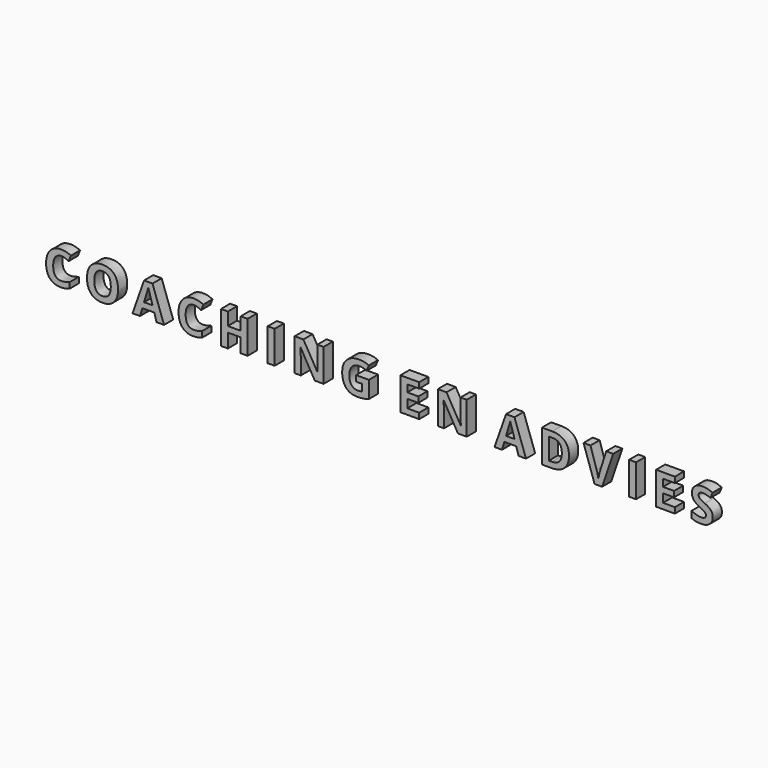
from build123d import *

# Parameters (mm, degrees)
F0_TEXT_SIZE = 79.5713910419
F1_DEPTH     = 20


# Not quite as in the source:
# - Text() gives the source's letters only with a copy of the font that has no kerning and outlines rounded to 1/6400 em; it was checked with that copy


with BuildPart() as f1:
    # F0 (on Front) → F1 (new body)
    with BuildSketch(Plane.XZ):
        with Locations((-60.2689087391, -13.0406077951)):
            Text('C O A C H I N G  E N  A D V I E S', F0_TEXT_SIZE, font='Open Sans', font_style=FontStyle.BOLD, text_align=(TextAlign.LEFT, TextAlign.BOTTOM))
    extrude(amount=F1_DEPTH)


solid = f1.part
